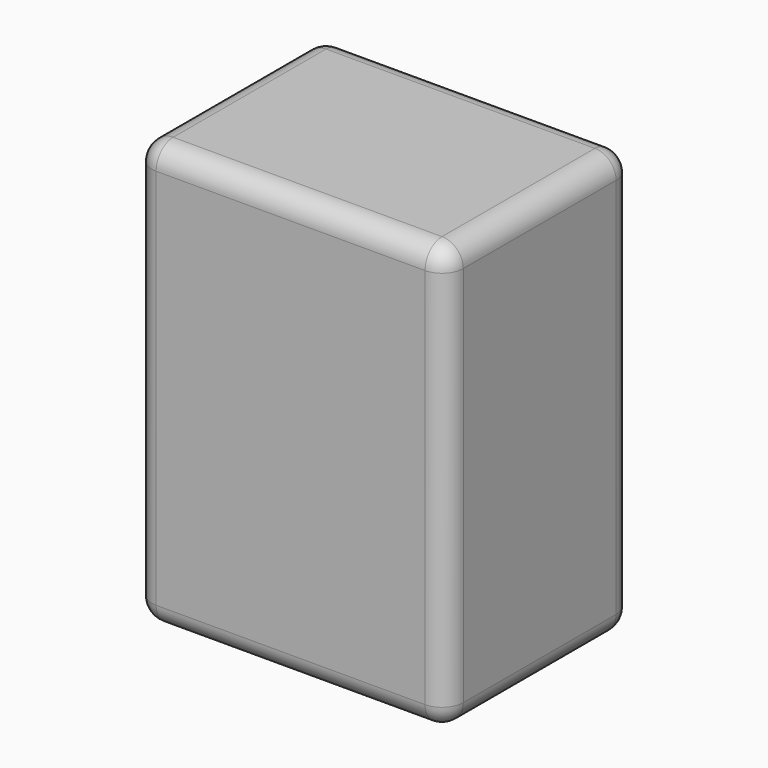
from build123d import *

# Parameters (mm, degrees)
F0_W     = 41
F0_H     = 33
F1_DEPTH = 60
F2_T     = -3
F3_W     = 27
F3_H     = 2
F4_DEPTH = 36
F5_W     = 33
F5_H     = 60
F6_DEPTH = 3
F7_W     = 27
F7_H     = 54
F7_W_2   = 25
F7_H_2   = 52
F8_DEPTH = 2
F9_R     = 3
F10_R    = 2.99999


# Not quite as in the source:
# - a fillet or chamfer is up to 0.001 mm smaller than in the source, because OpenCascade refuses the exact size


with BuildPart() as f1:
    # F0 (on Top) → F1 (new body)
    with BuildSketch(Plane.XY):
        with Locations((20.5, -16.5)):
            Rectangle(F0_W, F0_H)
    extrude(amount=F1_DEPTH)

    # F2
    f2_openings = [f1.faces().sort_by_distance(p)[0] for p in [
        (41, -16.5, 30),
    ]]
    offset(amount=F2_T, openings=f2_openings)

    # F3 (on face) → F4 (join)
    with BuildSketch(Plane.YZ.offset(3)):
        with Locations((-16.5, 38)):
            Rectangle(F3_W, F3_H)
    extrude(amount=F4_DEPTH)

    # F9
    f9_edges = [f1.edges().sort_by_distance(p)[0] for p in [
        (20.5, -33, 60),
        (20.5, 0, 60),
        (20.5, 0, 0),
        (20.5, -33, 0),
        (0, -33, 30),
        (0, -16.5, 60),
        (0, 0, 30),
        (0, -16.5, 0),
    ]]
    fillet(f9_edges, radius=F9_R)


with BuildPart() as f6:
    # F5 (on face) → F6 (new body)
    with BuildSketch(Plane.YZ.offset(41)):
        with Locations((-16.5, 30)):
            Rectangle(F5_W, F5_H)
    extrude(amount=F6_DEPTH)

    # F7 (on face) → F8 (join)
    with BuildSketch(Plane(origin=(41, 0, 0), x_dir=(0, -1, 0), z_dir=(-1, 0, 0))):
        with Locations((16.5, 30)):
            Rectangle(F7_W, F7_H)
        with Locations((16.5, 30)):
            Rectangle(F7_W_2, F7_H_2, mode=Mode.SUBTRACT)
    extrude(amount=F8_DEPTH)

    # F10 (radius 3 in the source; OpenCascade refuses exactly that, so slightly less here)
    f10_edges = [f6.edges().sort_by_distance(p)[0] for p in [
        (42.5, -33, 60),
        (44, -16.5, 60),
        (44, -33, 30),
        (44, -16.5, 0),
        (42.5, -33, 0),
        (42.5, 0, 0),
        (44, 0, 30),
        (42.5, 0, 60),
    ]]
    fillet(f10_edges, radius=F10_R)


solid = Compound([f1.part, f6.part])
